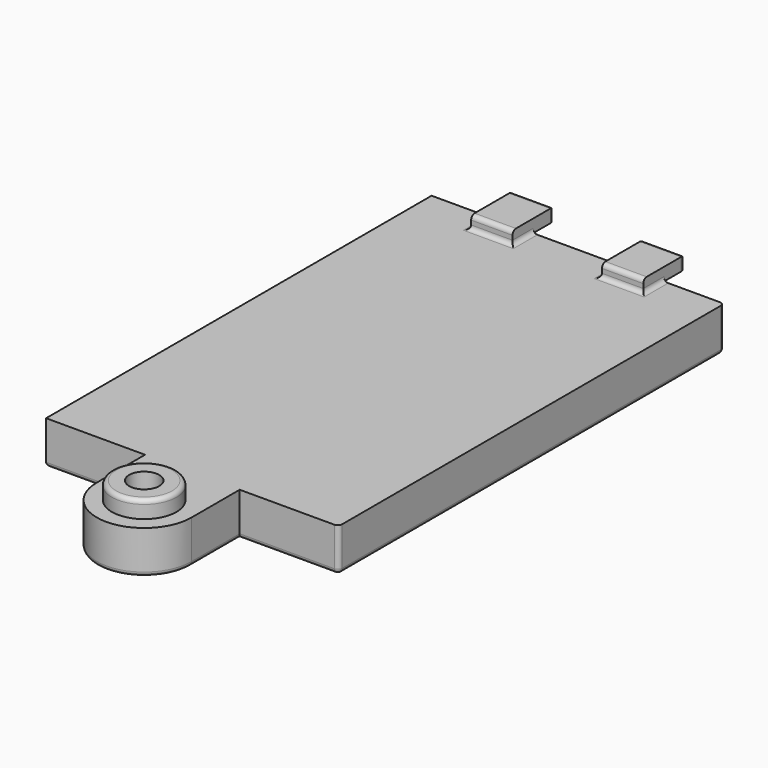
from build123d import *

# Parameters (mm, degrees)
F1_DEPTH = 5
F2_R     = 3.75
F3_DEPTH = 2
F4_D     = 3.5
F5_W     = 4.8
F5_H     = 6
F6_DEPTH = 1.5
F7_R     = 0.5


with BuildPart() as f1:
    # F0 (on Top) → F1 (new body)
    with BuildSketch(Plane.XY):
        Polygon((17, 29), (-17, 29), (-17, -27), (-5.5, -27), (5.5, -27), (17, -27), align=None)
        with BuildLine():
            Line((5.5, -27), (-5.5, -27))
            Line((-5.5, -27), (-5.5, -34))
            ThreePointArc((-5.5, -34), (0, -28.5), (5.5, -34))
            Line((5.5, -34), (5.5, -27))
        make_face()
        with BuildLine():
            ThreePointArc((5.5, -34), (0, -28.5), (-5.5, -34))
            ThreePointArc((-5.5, -34), (0, -39.5), (5.5, -34))
        make_face()
    extrude(amount=F1_DEPTH)

    # F2 (on face) → F3 (join)
    with BuildSketch(Plane.XY.offset(5)):
        with Locations((0, -34)):
            Circle(F2_R)
    extrude(amount=F3_DEPTH)

    # F4 (through all)
    with Locations(Plane(origin=(0, 0, 0), x_dir=(1, 0, 0), z_dir=(0, 0, -1))):
        with Locations((0, 34)):
            Hole(F4_D / 2)

    # F5 (on face) → F6 (join)
    with BuildSketch(Plane.XY.offset(5)):
        with Locations((-7.6, 29)):
            Rectangle(F5_W, F5_H)
        with Locations((7.6, 29)):
            Rectangle(F5_W, F5_H)
    extrude(amount=F6_DEPTH)

    # F7
    f7_edges = [f1.edges().sort_by_distance(p)[0] for p in [
        (7.6, 26, 6.5),
        (-7.6, 26, 6.5),
        (-7.6, 32, 6.5),
        (7.6, 32, 6.5),
        (0, 29, 0),
        (17, 29, 2.5),
        (17, 1, 0),
        (17, -27, 2.5),
        (5.5, -30.5, 0),
        (0, -39.5, 0),
        (-3.75, -34, 7),
        (11.25, -27, 0),
        (-11.25, -27, 0),
        (-17, 1, 0),
        (10, 32, 5.75),
        (5.2, 32, 5.75),
        (-5.2, 32, 5.75),
        (-10, 32, 5.75),
        (-7.6, 26, 5),
        (7.6, 26, 5),
        (5.2, 27.5, 5),
        (-10, 27.5, 5),
        (-5.2, 27.5, 5),
        (10, 27.5, 5),
        (-5.5, -30.5, 0),
    ]]
    fillet(f7_edges, radius=F7_R)


solid = f1.part
